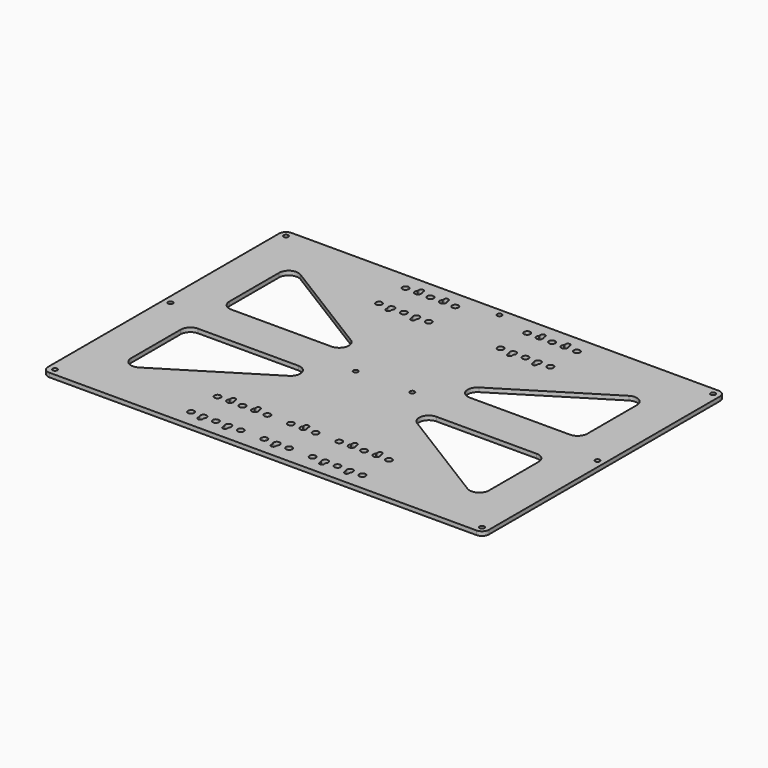
from build123d import *

# Parameters (mm, degrees)
F1_DEPTH = 3


# Not quite as in the source:
# - ends of sketch curves that miss each other by under 0.0002 mm in the source are joined


with BuildPart() as f1:
    # F0 (on Top) → F1 (new body)
    with BuildSketch(Plane.XY):
        with BuildLine():
            Line((62.37074, 242.018384), (62.37074, 33.018384))
            ThreePointArc((62.37074, 33.018384), (63.8352060941, 29.4828500941), (67.37074, 28.018384))
            Line((67.37074, 28.018384), (376.37074, 28.018384))
            ThreePointArc((376.37074, 28.018384), (379.9062739059, 29.4828500941), (381.37074, 33.018384))
            Line((381.37074, 33.018384), (381.37074, 242.018384))
            ThreePointArc((381.37074, 242.018384), (379.9062739059, 245.5539179059), (376.37074, 247.018384))
            Line((376.37074, 247.018384), (67.37074, 247.018384))
            ThreePointArc((67.37074, 247.018384), (63.8352060941, 245.5539179059), (62.37074, 242.018384))
        make_face()
        with BuildLine():
            ThreePointArc((67.37074, 34.718384), (68.572821528, 34.220465528), (69.07074, 33.018384))
            ThreePointArc((69.07074, 33.018384), (68.572821528, 31.816302472), (67.37074, 31.318384))
            ThreePointArc((67.37074, 31.318384), (66.168658472, 31.816302472), (65.67074, 33.018384))
            ThreePointArc((65.67074, 33.018384), (66.168658472, 34.220465528), (67.37074, 34.718384))
        make_face(mode=Mode.SUBTRACT)
        with BuildLine():
            ThreePointArc((159.87074, 42.768384), (161.4617302577, 42.1093742577), (162.12074, 40.518384))
            ThreePointArc((162.12074, 40.518384), (161.4617302577, 38.9273937423), (159.87074, 38.268384))
            ThreePointArc((159.87074, 38.268384), (158.2797497423, 38.9273937423), (157.62074, 40.518384))
            ThreePointArc((157.62074, 40.518384), (158.2797497423, 42.1093742577), (159.87074, 42.768384))
        make_face(mode=Mode.SUBTRACT)
        with BuildLine():
            ThreePointArc((170.47074, 37.518384), (168.87074, 35.918384), (167.27074, 37.518384))
            Line((167.27074, 37.518384), (167.27074, 38.936454))
            ThreePointArc((167.27074, 38.936454), (168.87074, 42.768384), (170.470739601, 38.9364543945))
            Line((170.470739601, 38.9364543945), (170.47074, 37.518384))
        make_face(mode=Mode.SUBTRACT)
        with BuildLine():
            ThreePointArc((177.87074, 42.768384), (179.4617302577, 42.1093742577), (180.12074, 40.518384))
            ThreePointArc((180.12074, 40.518384), (179.4617302577, 38.9273937423), (177.87074, 38.268384))
            ThreePointArc((177.87074, 38.268384), (176.2797497423, 38.9273937423), (175.62074, 40.518384))
            ThreePointArc((175.62074, 40.518384), (176.2797497423, 42.1093742577), (177.87074, 42.768384))
        make_face(mode=Mode.SUBTRACT)
        with BuildLine():
            ThreePointArc((188.47074, 37.518384), (186.87074, 35.918384), (185.27074, 37.518384))
            Line((185.27074, 37.518384), (185.27074, 38.936454))
            ThreePointArc((185.27074, 38.936454), (186.87074, 42.768384), (188.470739601, 38.9364543945))
            Line((188.470739601, 38.9364543945), (188.47074, 37.518384))
        make_face(mode=Mode.SUBTRACT)
        with BuildLine():
            ThreePointArc((195.87074, 42.768384), (197.4617302577, 42.1093742577), (198.12074, 40.518384))
            ThreePointArc((198.12074, 40.518384), (197.4617302577, 38.9273937423), (195.87074, 38.268384))
            ThreePointArc((195.87074, 38.268384), (194.2797497423, 38.9273937423), (193.62074, 40.518384))
            ThreePointArc((193.62074, 40.518384), (194.2797497423, 42.1093742577), (195.87074, 42.768384))
        make_face(mode=Mode.SUBTRACT)
        with BuildLine():
            ThreePointArc((212.87074, 42.768384), (214.4617302577, 42.1093742577), (215.12074, 40.518384))
            ThreePointArc((215.12074, 40.518384), (214.4617302577, 38.9273937423), (212.87074, 38.268384))
            ThreePointArc((212.87074, 38.268384), (211.2797497423, 38.9273937423), (210.62074, 40.518384))
            ThreePointArc((210.62074, 40.518384), (211.2797497423, 42.1093742577), (212.87074, 42.768384))
        make_face(mode=Mode.SUBTRACT)
        with BuildLine():
            ThreePointArc((159.87074, 66.768384), (161.4617302577, 66.1093742577), (162.12074, 64.518384))
            ThreePointArc((162.12074, 64.518384), (161.4617302577, 62.9273937423), (159.87074, 62.268384))
            ThreePointArc((159.87074, 62.268384), (158.2797497423, 62.9273937423), (157.62074, 64.518384))
            ThreePointArc((157.62074, 64.518384), (158.2797497423, 66.1093742577), (159.87074, 66.768384))
        make_face(mode=Mode.SUBTRACT)
        with BuildLine():
            ThreePointArc((167.27074, 67.518384), (168.87074, 69.118384), (170.47074, 67.518384))
            Line((170.47074, 67.518384), (170.47074, 66.100313))
            ThreePointArc((170.47074, 66.100313), (168.87074, 62.268384), (167.270739899, 66.1003130998))
            Line((167.270739899, 66.1003130998), (167.27074, 67.518384))
        make_face(mode=Mode.SUBTRACT)
        with BuildLine():
            ThreePointArc((177.87074, 66.768384), (179.4617302577, 66.1093742577), (180.12074, 64.518384))
            ThreePointArc((180.12074, 64.518384), (179.4617302577, 62.9273937423), (177.87074, 62.268384))
            ThreePointArc((177.87074, 62.268384), (176.2797497423, 62.9273937423), (175.62074, 64.518384))
            ThreePointArc((175.62074, 64.518384), (176.2797497423, 66.1093742577), (177.87074, 66.768384))
        make_face(mode=Mode.SUBTRACT)
        with BuildLine():
            ThreePointArc((185.27074, 67.518384), (186.87074, 69.118384), (188.47074, 67.518384))
            Line((188.47074, 67.518384), (188.47074, 66.100313))
            ThreePointArc((188.47074, 66.100313), (186.87074, 62.268384), (185.270739899, 66.1003130998))
            Line((185.270739899, 66.1003130998), (185.27074, 67.518384))
        make_face(mode=Mode.SUBTRACT)
        with BuildLine():
            ThreePointArc((195.87074, 66.768384), (197.4617302577, 66.1093742577), (198.12074, 64.518384))
            ThreePointArc((198.12074, 64.518384), (197.4617302577, 62.9273937423), (195.87074, 62.268384))
            ThreePointArc((195.87074, 62.268384), (194.2797497423, 62.9273937423), (193.62074, 64.518384))
            ThreePointArc((193.62074, 64.518384), (194.2797497423, 66.1093742577), (195.87074, 66.768384))
        make_face(mode=Mode.SUBTRACT)
        with BuildLine():
            ThreePointArc((212.87074, 66.768384), (214.4617302577, 66.1093742577), (215.12074, 64.518384))
            ThreePointArc((215.12074, 64.518384), (214.4617302577, 62.9273937423), (212.87074, 62.268384))
            ThreePointArc((212.87074, 62.268384), (211.2797497423, 62.9273937423), (210.62074, 64.518384))
            ThreePointArc((210.62074, 64.518384), (211.2797497423, 66.1093742577), (212.87074, 66.768384))
        make_face(mode=Mode.SUBTRACT)
        with BuildLine():
            Line((99.37074, 122.518384), (171.87074, 122.518384))
            ThreePointArc((171.87074, 122.518384), (178.603165852, 117.4352674464), (175.5579616199, 109.5682246134))
            Line((175.5579616199, 109.5682246134), (103.057962, 64.641091))
            ThreePointArc((103.057962, 64.641091), (95.96563754, 64.4752646144), (92.37074, 70.59125))
            Line((92.37074, 70.59125), (92.37074, 115.518384))
            ThreePointArc((92.37074, 115.518384), (94.4209925317, 120.4681314683), (99.37074, 122.518384))
        make_face(mode=Mode.SUBTRACT)
        with BuildLine():
            ThreePointArc((223.47074, 37.518384), (221.87074, 35.918384), (220.27074, 37.518384))
            Line((220.27074, 37.518384), (220.27074, 38.936454))
            ThreePointArc((220.27074, 38.936454), (221.87074, 42.768384), (223.470739601, 38.9364543945))
            Line((223.470739601, 38.9364543945), (223.47074, 37.518384))
        make_face(mode=Mode.SUBTRACT)
        with BuildLine():
            ThreePointArc((230.87074, 42.768384), (232.4617302577, 42.1093742577), (233.12074, 40.518384))
            ThreePointArc((233.12074, 40.518384), (232.4617302577, 38.9273937423), (230.87074, 38.268384))
            ThreePointArc((230.87074, 38.268384), (229.2797497423, 38.9273937423), (228.62074, 40.518384))
            ThreePointArc((228.62074, 40.518384), (229.2797497423, 42.1093742577), (230.87074, 42.768384))
        make_face(mode=Mode.SUBTRACT)
        with BuildLine():
            ThreePointArc((247.87074, 42.768384), (249.4617302577, 42.1093742577), (250.12074, 40.518384))
            ThreePointArc((250.12074, 40.518384), (249.4617302577, 38.9273937423), (247.87074, 38.268384))
            ThreePointArc((247.87074, 38.268384), (246.2797497423, 38.9273937423), (245.62074, 40.518384))
            ThreePointArc((245.62074, 40.518384), (246.2797497423, 42.1093742577), (247.87074, 42.768384))
        make_face(mode=Mode.SUBTRACT)
        with BuildLine():
            ThreePointArc((258.47074, 37.518384), (256.87074, 35.918384), (255.27074, 37.518384))
            Line((255.27074, 37.518384), (255.27074, 38.936454))
            ThreePointArc((255.27074, 38.936454), (256.87074, 42.768384), (258.470739601, 38.9364543945))
            Line((258.470739601, 38.9364543945), (258.47074, 37.518384))
        make_face(mode=Mode.SUBTRACT)
        with BuildLine():
            ThreePointArc((265.87074, 42.768384), (267.4617302577, 42.1093742577), (268.12074, 40.518384))
            ThreePointArc((268.12074, 40.518384), (267.4617302577, 38.9273937423), (265.87074, 38.268384))
            ThreePointArc((265.87074, 38.268384), (264.2797497423, 38.9273937423), (263.62074, 40.518384))
            ThreePointArc((263.62074, 40.518384), (264.2797497423, 42.1093742577), (265.87074, 42.768384))
        make_face(mode=Mode.SUBTRACT)
        with BuildLine():
            ThreePointArc((276.47074, 37.518384), (274.87074, 35.918384), (273.27074, 37.518384))
            Line((273.27074, 37.518384), (273.27074, 38.936454))
            ThreePointArc((273.27074, 38.936454), (274.87074, 42.768384), (276.470739601, 38.9364543945))
            Line((276.470739601, 38.9364543945), (276.47074, 37.518384))
        make_face(mode=Mode.SUBTRACT)
        with BuildLine():
            ThreePointArc((283.87074, 42.768384), (285.4617302577, 42.1093742577), (286.12074, 40.518384))
            ThreePointArc((286.12074, 40.518384), (285.4617302577, 38.9273937423), (283.87074, 38.268384))
            ThreePointArc((283.87074, 38.268384), (282.2797497423, 38.9273937423), (281.62074, 40.518384))
            ThreePointArc((281.62074, 40.518384), (282.2797497423, 42.1093742577), (283.87074, 42.768384))
        make_face(mode=Mode.SUBTRACT)
        with BuildLine():
            ThreePointArc((230.87074, 66.768384), (232.4617302577, 66.1093742577), (233.12074, 64.518384))
            ThreePointArc((233.12074, 64.518384), (232.4617302577, 62.9273937423), (230.87074, 62.268384))
            ThreePointArc((230.87074, 62.268384), (229.2797497423, 62.9273937423), (228.62074, 64.518384))
            ThreePointArc((228.62074, 64.518384), (229.2797497423, 66.1093742577), (230.87074, 66.768384))
        make_face(mode=Mode.SUBTRACT)
        with BuildLine():
            ThreePointArc((220.27074, 67.518384), (221.87074, 69.118384), (223.47074, 67.518384))
            Line((223.47074, 67.518384), (223.47074, 66.100313))
            ThreePointArc((223.47074, 66.100313), (221.87074, 62.268384), (220.270739899, 66.1003130998))
            Line((220.270739899, 66.1003130998), (220.27074, 67.518384))
        make_face(mode=Mode.SUBTRACT)
        with BuildLine():
            ThreePointArc((247.87074, 66.768384), (249.4617302577, 66.1093742577), (250.12074, 64.518384))
            ThreePointArc((250.12074, 64.518384), (249.4617302577, 62.9273937423), (247.87074, 62.268384))
            ThreePointArc((247.87074, 62.268384), (246.2797497423, 62.9273937423), (245.62074, 64.518384))
            ThreePointArc((245.62074, 64.518384), (246.2797497423, 66.1093742577), (247.87074, 66.768384))
        make_face(mode=Mode.SUBTRACT)
        with BuildLine():
            ThreePointArc((255.27074, 67.518384), (256.87074, 69.118384), (258.47074, 67.518384))
            Line((258.47074, 67.518384), (258.47074, 66.100313))
            ThreePointArc((258.47074, 66.100313), (256.87074, 62.268384), (255.270739899, 66.1003130998))
            Line((255.270739899, 66.1003130998), (255.27074, 67.518384))
        make_face(mode=Mode.SUBTRACT)
        with BuildLine():
            ThreePointArc((265.87074, 66.768384), (267.4617302577, 66.1093742577), (268.12074, 64.518384))
            ThreePointArc((268.12074, 64.518384), (267.4617302577, 62.9273937423), (265.87074, 62.268384))
            ThreePointArc((265.87074, 62.268384), (264.2797497423, 62.9273937423), (263.62074, 64.518384))
            ThreePointArc((263.62074, 64.518384), (264.2797497423, 66.1093742577), (265.87074, 66.768384))
        make_face(mode=Mode.SUBTRACT)
        with BuildLine():
            ThreePointArc((273.27074, 67.518384), (274.87074, 69.118384), (276.47074, 67.518384))
            Line((276.47074, 67.518384), (276.47074, 66.100313))
            ThreePointArc((276.47074, 66.100313), (274.87074, 62.268384), (273.270739899, 66.1003130998))
            Line((273.270739899, 66.1003130998), (273.27074, 67.518384))
        make_face(mode=Mode.SUBTRACT)
        with BuildLine():
            ThreePointArc((283.87074, 66.768384), (285.4617302577, 66.1093742577), (286.12074, 64.518384))
            ThreePointArc((286.12074, 64.518384), (285.4617302577, 62.9273937423), (283.87074, 62.268384))
            ThreePointArc((283.87074, 62.268384), (282.2797497423, 62.9273937423), (281.62074, 64.518384))
            ThreePointArc((281.62074, 64.518384), (282.2797497423, 66.1093742577), (283.87074, 66.768384))
        make_face(mode=Mode.SUBTRACT)
        with BuildLine():
            ThreePointArc((376.37074, 34.718384), (377.572821528, 34.220465528), (378.07074, 33.018384))
            ThreePointArc((378.07074, 33.018384), (377.572821528, 31.816302472), (376.37074, 31.318384))
            ThreePointArc((376.37074, 31.318384), (375.168658472, 31.816302472), (374.67074, 33.018384))
            ThreePointArc((374.67074, 33.018384), (375.168658472, 34.220465528), (376.37074, 34.718384))
        make_face(mode=Mode.SUBTRACT)
        with BuildLine():
            Line((351.37074, 115.518384), (351.37074, 70.59125))
            ThreePointArc((351.37074, 70.59125), (347.77584246, 64.4752646144), (340.6835179324, 64.6410908909))
            Line((340.6835179324, 64.6410908909), (268.183518, 109.568224))
            ThreePointArc((268.183518, 109.568224), (265.138314148, 117.4352674464), (271.87074, 122.518384))
            Line((271.87074, 122.518384), (344.37074, 122.518384))
            ThreePointArc((344.37074, 122.518384), (349.3204874683, 120.4681314683), (351.37074, 115.518384))
        make_face(mode=Mode.SUBTRACT)
        with BuildLine():
            ThreePointArc((67.37074, 139.218384), (68.572821528, 138.720465528), (69.07074, 137.518384))
            ThreePointArc((69.07074, 137.518384), (68.572821528, 136.316302472), (67.37074, 135.818384))
            ThreePointArc((67.37074, 135.818384), (66.168658472, 136.316302472), (65.67074, 137.518384))
            ThreePointArc((65.67074, 137.518384), (66.168658472, 138.720465528), (67.37074, 139.218384))
        make_face(mode=Mode.SUBTRACT)
        with BuildLine():
            Line((92.37074, 159.518384), (92.37074, 204.445517))
            ThreePointArc((92.37074, 204.445517), (95.9656373099, 210.5615022575), (103.0579616199, 210.3956763866))
            Line((103.0579616199, 210.3956763866), (175.557962, 165.468543))
            ThreePointArc((175.557962, 165.468543), (178.6031657799, 157.6015003003), (171.87074, 152.518384))
            Line((171.87074, 152.518384), (99.37074, 152.518384))
            ThreePointArc((99.37074, 152.518384), (94.4209925317, 154.5686365317), (92.37074, 159.518384))
        make_face(mode=Mode.SUBTRACT)
        with BuildLine():
            ThreePointArc((201.37074, 139.218384), (202.572821528, 138.720465528), (203.07074, 137.518384))
            ThreePointArc((203.07074, 137.518384), (202.572821528, 136.316302472), (201.37074, 135.818384))
            ThreePointArc((201.37074, 135.818384), (200.168658472, 136.316302472), (199.67074, 137.518384))
            ThreePointArc((199.67074, 137.518384), (200.168658472, 138.720465528), (201.37074, 139.218384))
        make_face(mode=Mode.SUBTRACT)
        with BuildLine():
            ThreePointArc((67.37074, 243.718384), (68.572821528, 243.220465528), (69.07074, 242.018384))
            ThreePointArc((69.07074, 242.018384), (68.572821528, 240.816302472), (67.37074, 240.318384))
            ThreePointArc((67.37074, 240.318384), (66.168658472, 240.816302472), (65.67074, 242.018384))
            ThreePointArc((65.67074, 242.018384), (66.168658472, 243.220465528), (67.37074, 243.718384))
        make_face(mode=Mode.SUBTRACT)
        with BuildLine():
            ThreePointArc((159.87074, 212.768384), (161.4617302577, 212.1093742577), (162.12074, 210.518384))
            ThreePointArc((162.12074, 210.518384), (161.4617302577, 208.9273937423), (159.87074, 208.268384))
            ThreePointArc((159.87074, 208.268384), (158.2797497423, 208.9273937423), (157.62074, 210.518384))
            ThreePointArc((157.62074, 210.518384), (158.2797497423, 212.1093742577), (159.87074, 212.768384))
        make_face(mode=Mode.SUBTRACT)
        with BuildLine():
            ThreePointArc((167.270740399, 208.9364543945), (168.87074, 212.768384), (170.470739601, 208.9364543945))
            Line((170.470739601, 208.9364543945), (170.47074, 207.518384))
            ThreePointArc((170.47074, 207.518384), (168.87074, 205.918384), (167.27074, 207.518384))
            Line((167.27074, 207.518384), (167.270740399, 208.9364543945))
        make_face(mode=Mode.SUBTRACT)
        with BuildLine():
            ThreePointArc((177.87074, 212.768384), (179.4617302577, 212.1093742577), (180.12074, 210.518384))
            ThreePointArc((180.12074, 210.518384), (179.4617302577, 208.9273937423), (177.87074, 208.268384))
            ThreePointArc((177.87074, 208.268384), (176.2797497423, 208.9273937423), (175.62074, 210.518384))
            ThreePointArc((175.62074, 210.518384), (176.2797497423, 212.1093742577), (177.87074, 212.768384))
        make_face(mode=Mode.SUBTRACT)
        with BuildLine():
            ThreePointArc((185.270740399, 208.9364543945), (186.87074, 212.768384), (188.470739601, 208.9364543945))
            Line((188.470739601, 208.9364543945), (188.47074, 207.518384))
            ThreePointArc((188.47074, 207.518384), (186.87074, 205.918384), (185.27074, 207.518384))
            Line((185.27074, 207.518384), (185.270740399, 208.9364543945))
        make_face(mode=Mode.SUBTRACT)
        with BuildLine():
            ThreePointArc((195.87074, 212.768384), (197.4617302577, 212.1093742577), (198.12074, 210.518384))
            ThreePointArc((198.12074, 210.518384), (197.4617302577, 208.9273937423), (195.87074, 208.268384))
            ThreePointArc((195.87074, 208.268384), (194.2797497423, 208.9273937423), (193.62074, 210.518384))
            ThreePointArc((193.62074, 210.518384), (194.2797497423, 212.1093742577), (195.87074, 212.768384))
        make_face(mode=Mode.SUBTRACT)
        with BuildLine():
            ThreePointArc((159.87074, 236.768384), (161.4617302577, 236.1093742577), (162.12074, 234.518384))
            ThreePointArc((162.12074, 234.518384), (161.4617302577, 232.9273937423), (159.87074, 232.268384))
            ThreePointArc((159.87074, 232.268384), (158.2797497423, 232.9273937423), (157.62074, 234.518384))
            ThreePointArc((157.62074, 234.518384), (158.2797497423, 236.1093742577), (159.87074, 236.768384))
        make_face(mode=Mode.SUBTRACT)
        with BuildLine():
            ThreePointArc((170.470740101, 236.1003130998), (168.87074, 232.268384), (167.270739899, 236.1003130998))
            Line((167.270739899, 236.1003130998), (167.27074, 237.518384))
            ThreePointArc((167.27074, 237.518384), (168.87074, 239.118384), (170.47074, 237.518384))
            Line((170.47074, 237.518384), (170.470740101, 236.1003130998))
        make_face(mode=Mode.SUBTRACT)
        with BuildLine():
            ThreePointArc((177.87074, 236.768384), (179.4617302577, 236.1093742577), (180.12074, 234.518384))
            ThreePointArc((180.12074, 234.518384), (179.4617302577, 232.9273937423), (177.87074, 232.268384))
            ThreePointArc((177.87074, 232.268384), (176.2797497423, 232.9273937423), (175.62074, 234.518384))
            ThreePointArc((175.62074, 234.518384), (176.2797497423, 236.1093742577), (177.87074, 236.768384))
        make_face(mode=Mode.SUBTRACT)
        with BuildLine():
            ThreePointArc((188.470740101, 236.1003130998), (186.87074, 232.268384), (185.270739899, 236.1003130998))
            Line((185.270739899, 236.1003130998), (185.27074, 237.518384))
            ThreePointArc((185.27074, 237.518384), (186.87074, 239.118384), (188.47074, 237.518384))
            Line((188.47074, 237.518384), (188.470740101, 236.1003130998))
        make_face(mode=Mode.SUBTRACT)
        with BuildLine():
            ThreePointArc((195.87074, 236.768384), (197.4617302577, 236.1093742577), (198.12074, 234.518384))
            ThreePointArc((198.12074, 234.518384), (197.4617302577, 232.9273937423), (195.87074, 232.268384))
            ThreePointArc((195.87074, 232.268384), (194.2797497423, 232.9273937423), (193.62074, 234.518384))
            ThreePointArc((193.62074, 234.518384), (194.2797497423, 236.1093742577), (195.87074, 236.768384))
        make_face(mode=Mode.SUBTRACT)
        with BuildLine():
            ThreePointArc((242.37074, 139.218384), (243.572821528, 138.720465528), (244.07074, 137.518384))
            ThreePointArc((244.07074, 137.518384), (243.572821528, 136.316302472), (242.37074, 135.818384))
            ThreePointArc((242.37074, 135.818384), (241.168658472, 136.316302472), (240.67074, 137.518384))
            ThreePointArc((240.67074, 137.518384), (241.168658472, 138.720465528), (242.37074, 139.218384))
        make_face(mode=Mode.SUBTRACT)
        with BuildLine():
            ThreePointArc((376.37074, 139.218384), (377.572821528, 138.720465528), (378.07074, 137.518384))
            ThreePointArc((378.07074, 137.518384), (377.572821528, 136.316302472), (376.37074, 135.818384))
            ThreePointArc((376.37074, 135.818384), (375.168658472, 136.316302472), (374.67074, 137.518384))
            ThreePointArc((374.67074, 137.518384), (375.168658472, 138.720465528), (376.37074, 139.218384))
        make_face(mode=Mode.SUBTRACT)
        with BuildLine():
            Line((344.37074, 152.518384), (271.87074, 152.518384))
            ThreePointArc((271.87074, 152.518384), (265.1383142201, 157.6015003003), (268.1835179324, 165.4685431091))
            Line((268.1835179324, 165.4685431091), (340.683518, 210.395677))
            ThreePointArc((340.683518, 210.395677), (347.7758426901, 210.5615022575), (351.37074, 204.445517))
            Line((351.37074, 204.445517), (351.37074, 159.518384))
            ThreePointArc((351.37074, 159.518384), (349.3204874683, 154.5686365317), (344.37074, 152.518384))
        make_face(mode=Mode.SUBTRACT)
        with BuildLine():
            ThreePointArc((247.87074, 212.768384), (249.4617302577, 212.1093742577), (250.12074, 210.518384))
            ThreePointArc((250.12074, 210.518384), (249.4617302577, 208.9273937423), (247.87074, 208.268384))
            ThreePointArc((247.87074, 208.268384), (246.2797497423, 208.9273937423), (245.62074, 210.518384))
            ThreePointArc((245.62074, 210.518384), (246.2797497423, 212.1093742577), (247.87074, 212.768384))
        make_face(mode=Mode.SUBTRACT)
        with BuildLine():
            ThreePointArc((255.270740399, 208.9364543945), (256.87074, 212.768384), (258.470739601, 208.9364543945))
            Line((258.470739601, 208.9364543945), (258.47074, 207.518384))
            ThreePointArc((258.47074, 207.518384), (256.87074, 205.918384), (255.27074, 207.518384))
            Line((255.27074, 207.518384), (255.270740399, 208.9364543945))
        make_face(mode=Mode.SUBTRACT)
        with BuildLine():
            ThreePointArc((265.87074, 212.768384), (267.4617302577, 212.1093742577), (268.12074, 210.518384))
            ThreePointArc((268.12074, 210.518384), (267.4617302577, 208.9273937423), (265.87074, 208.268384))
            ThreePointArc((265.87074, 208.268384), (264.2797497423, 208.9273937423), (263.62074, 210.518384))
            ThreePointArc((263.62074, 210.518384), (264.2797497423, 212.1093742577), (265.87074, 212.768384))
        make_face(mode=Mode.SUBTRACT)
        with BuildLine():
            ThreePointArc((273.270740399, 208.9364543945), (274.87074, 212.768384), (276.470739601, 208.9364543945))
            Line((276.470739601, 208.9364543945), (276.47074, 207.518384))
            ThreePointArc((276.47074, 207.518384), (274.87074, 205.918384), (273.27074, 207.518384))
            Line((273.27074, 207.518384), (273.270740399, 208.9364543945))
        make_face(mode=Mode.SUBTRACT)
        with BuildLine():
            ThreePointArc((283.87074, 212.768384), (285.4617302577, 212.1093742577), (286.12074, 210.518384))
            ThreePointArc((286.12074, 210.518384), (285.4617302577, 208.9273937423), (283.87074, 208.268384))
            ThreePointArc((283.87074, 208.268384), (282.2797497423, 208.9273937423), (281.62074, 210.518384))
            ThreePointArc((281.62074, 210.518384), (282.2797497423, 212.1093742577), (283.87074, 212.768384))
        make_face(mode=Mode.SUBTRACT)
        with BuildLine():
            ThreePointArc((221.87074, 243.718384), (223.072821528, 243.220465528), (223.57074, 242.018384))
            ThreePointArc((223.57074, 242.018384), (223.072821528, 240.816302472), (221.87074, 240.318384))
            ThreePointArc((221.87074, 240.318384), (220.668658472, 240.816302472), (220.17074, 242.018384))
            ThreePointArc((220.17074, 242.018384), (220.668658472, 243.220465528), (221.87074, 243.718384))
        make_face(mode=Mode.SUBTRACT)
        with BuildLine():
            ThreePointArc((247.87074, 236.768384), (249.4617302577, 236.1093742577), (250.12074, 234.518384))
            ThreePointArc((250.12074, 234.518384), (249.4617302577, 232.9273937423), (247.87074, 232.268384))
            ThreePointArc((247.87074, 232.268384), (246.2797497423, 232.9273937423), (245.62074, 234.518384))
            ThreePointArc((245.62074, 234.518384), (246.2797497423, 236.1093742577), (247.87074, 236.768384))
        make_face(mode=Mode.SUBTRACT)
        with BuildLine():
            ThreePointArc((258.470740101, 236.1003130998), (256.87074, 232.268384), (255.270739899, 236.1003130998))
            Line((255.270739899, 236.1003130998), (255.27074, 237.518384))
            ThreePointArc((255.27074, 237.518384), (256.87074, 239.118384), (258.47074, 237.518384))
            Line((258.47074, 237.518384), (258.470740101, 236.1003130998))
        make_face(mode=Mode.SUBTRACT)
        with BuildLine():
            ThreePointArc((265.87074, 236.768384), (267.4617302577, 236.1093742577), (268.12074, 234.518384))
            ThreePointArc((268.12074, 234.518384), (267.4617302577, 232.9273937423), (265.87074, 232.268384))
            ThreePointArc((265.87074, 232.268384), (264.2797497423, 232.9273937423), (263.62074, 234.518384))
            ThreePointArc((263.62074, 234.518384), (264.2797497423, 236.1093742577), (265.87074, 236.768384))
        make_face(mode=Mode.SUBTRACT)
        with BuildLine():
            ThreePointArc((276.470740101, 236.1003130998), (274.87074, 232.268384), (273.270739899, 236.1003130998))
            Line((273.270739899, 236.1003130998), (273.27074, 237.518384))
            ThreePointArc((273.27074, 237.518384), (274.87074, 239.118384), (276.47074, 237.518384))
            Line((276.47074, 237.518384), (276.470740101, 236.1003130998))
        make_face(mode=Mode.SUBTRACT)
        with BuildLine():
            ThreePointArc((283.87074, 236.768384), (285.4617302577, 236.1093742577), (286.12074, 234.518384))
            ThreePointArc((286.12074, 234.518384), (285.4617302577, 232.9273937423), (283.87074, 232.268384))
            ThreePointArc((283.87074, 232.268384), (282.2797497423, 232.9273937423), (281.62074, 234.518384))
            ThreePointArc((281.62074, 234.518384), (282.2797497423, 236.1093742577), (283.87074, 236.768384))
        make_face(mode=Mode.SUBTRACT)
        with BuildLine():
            ThreePointArc((376.37074, 243.718384), (377.572821528, 243.220465528), (378.07074, 242.018384))
            ThreePointArc((378.07074, 242.018384), (377.572821528, 240.816302472), (376.37074, 240.318384))
            ThreePointArc((376.37074, 240.318384), (375.168658472, 240.816302472), (374.67074, 242.018384))
            ThreePointArc((374.67074, 242.018384), (375.168658472, 243.220465528), (376.37074, 243.718384))
        make_face(mode=Mode.SUBTRACT)
    extrude(amount=F1_DEPTH)


solid = f1.part
